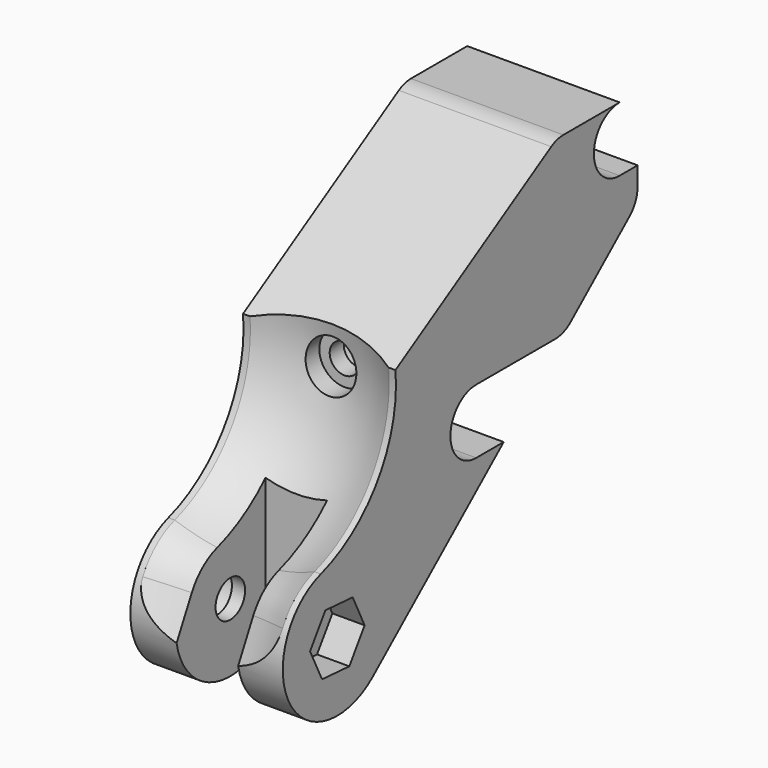
from build123d import *

# Parameters (mm, degrees)
F0_R      = 3.15
F1_DEPTH  = 13
F3_DEPTH  = 5.25
F5_DEPTH  = 5.5
F6_R      = 5.05
F7_DEPTH  = 5.5
F13_ANGLE = 45
F14_DEPTH = 15.67431457


# Not quite as in the source:
# - ends of sketch curves that miss each other by under 0.0002 mm in the source are joined


with BuildPart() as f1:
    # F0 (on Right) → F1 (new body, symmetric)
    with BuildSketch(Plane.YZ):
        with BuildLine():
            ThreePointArc((0.206929, -7.128644), (-5.293071, -1.628644), (0.206929, 3.871356))
            Line((0.206929, 3.871356), (17.0618508568, 3.871356))
            ThreePointArc((17.0618508568, 3.871356), (18.7952856408, 4.1814515394), (20.3137082671, 5.0732744602))
            Line((20.3137082671, 5.0732744602), (32.8624566897, 15.8173146076))
            ThreePointArc((32.8624566897, 15.8173146076), (34.1525860171, 17.5248563908), (34.6105992794, 19.6153961475))
            Line((34.6105992794, 19.6153961475), (34.6105992794, 22.815095))
            Line((34.6105992794, 22.815095), (30.788173, 22.815095))
            ThreePointArc((30.788173, 22.815095), (25.288173, 28.315095), (30.788173, 33.815095))
            Line((30.788173, 33.815095), (18.7829781294, 33.815095))
            ThreePointArc((18.7829781294, 33.815095), (17.4423484261, 33.6320143473), (16.1998960673, 33.0961797995))
            Line((16.1998960673, 33.0961797995), (-17.01485, 13.055368))
            ThreePointArc((-17.01485, 13.055368), (-20.6995911511, -1.839295663), (-32.9318010984, -11.1021976908))
            ThreePointArc((-32.9318010984, -11.1021976908), (-39.5666476125, -27.8428278397), (-21.8415422013, -31.0193857649))
            Line((-21.8415422013, -31.0193857649), (6.062198, -7.128644))
            Line((6.062198, -7.128644), (0.206929, -7.128644))
        make_face()
        with Locations((-29.405486, -22.184905)):
            Circle(F0_R, mode=Mode.SUBTRACT)
    extrude(amount=F1_DEPTH, both=True)

    # F2 (on Right) → F3 (cut, symmetric)
    with BuildSketch(Plane.YZ):
        with BuildLine():
            ThreePointArc((-21.905486, -3.502726), (-26.8533127567, -8.1227182817), (-32.9318011292, -11.1021976663))
            ThreePointArc((-32.9318011292, -11.1021976663), (-39.5869945241, -27.806130876), (-21.905486, -31.0737348541))
            Line((-21.905486, -31.0737348541), (-21.905486, -3.502726))
        make_face()
    extrude(amount=F3_DEPTH, both=True, mode=Mode.SUBTRACT)

    # F4 (on face) → F5 (cut)
    with BuildSketch(Plane.YZ.offset(13)):
        Polygon((-26.8555401867, -27.4290550439), (-23.5889459341, -22.5986621693), (-26.1388917474, -17.3545121255), (-31.9554318133, -16.9407549561), (-35.2220260659, -21.7711478307), (-32.6720802526, -27.0152978745), align=None)
    extrude(amount=-F5_DEPTH, mode=Mode.SUBTRACT)

    # F6 (on face) → F7 (cut)
    with BuildSketch(Plane(origin=(-13, 0, 0), x_dir=(0, -1, 0), z_dir=(-1, 0, 0))):
        with Locations((29.405486, -22.184905)):
            Circle(F6_R)
    extrude(amount=-F7_DEPTH, mode=Mode.SUBTRACT)

    # F8 (on Right) → F9 (revolve, cut)
    with BuildSketch(Plane.YZ):
        Polygon((30.9979878552, 13.8976717895), (-8.6011026711, 13.8976717895), (-8.6011026711, 10.921356), (-11.6011026711, 10.921356), (-11.6011026711, 12.6871454737), (-20.2870493605, 12.6871454737), (-20.375526354, 8.371356), (30.9979878552, 8.371356), align=None)
    revolve(axis=Axis((0, 5.3112307506, 8.371356), (0, -1, 0)), mode=Mode.SUBTRACT)

    # F11 (on 3pt) → F12 (revolve, cut)
    with BuildSketch(Plane(origin=(0, -33.1120649043, -10.535657015), x_dir=(-1, 0, 0), z_dir=(0, 0.95292578, 0.3032036573))):
        with BuildLine():
            Line((13, 0), (-13, 0))
            ThreePointArc((-13, 0), (0, -3.5066758251), (13, 0))
        make_face()
    revolve(axis=Axis((6.7580873147, -39.8867132027, 10.75609478), (1, 0, 0)), mode=Mode.SUBTRACT)

    # F11 (on 3pt) → F13 (revolve, cut)
    with BuildSketch(Plane(origin=(0, -33.1120649043, -10.535657015), x_dir=(-1, 0, 0), z_dir=(0, 0.95292578, 0.3032036573))):
        with BuildLine():
            Line((13, 0), (-13, 0))
            ThreePointArc((-13, 0), (0, -3.5066758251), (13, 0))
        make_face()
    revolve(axis=Axis((6.5, -29.405486, -22.184905), (1, 0, 0)), revolution_arc=F13_ANGLE, mode=Mode.SUBTRACT)

    # F14 (cut, through all): faces of the model
    f14_faces = [f1.faces().sort_by_distance(p)[0] for p in [
        (-7.6184233171, -38.9779934398, -17.2336080484),
        (7.6184233311, -38.9779934508, -17.2336080427),
    ]]
    extrude(f14_faces, amount=-F14_DEPTH, mode=Mode.SUBTRACT)


solid = f1.part
